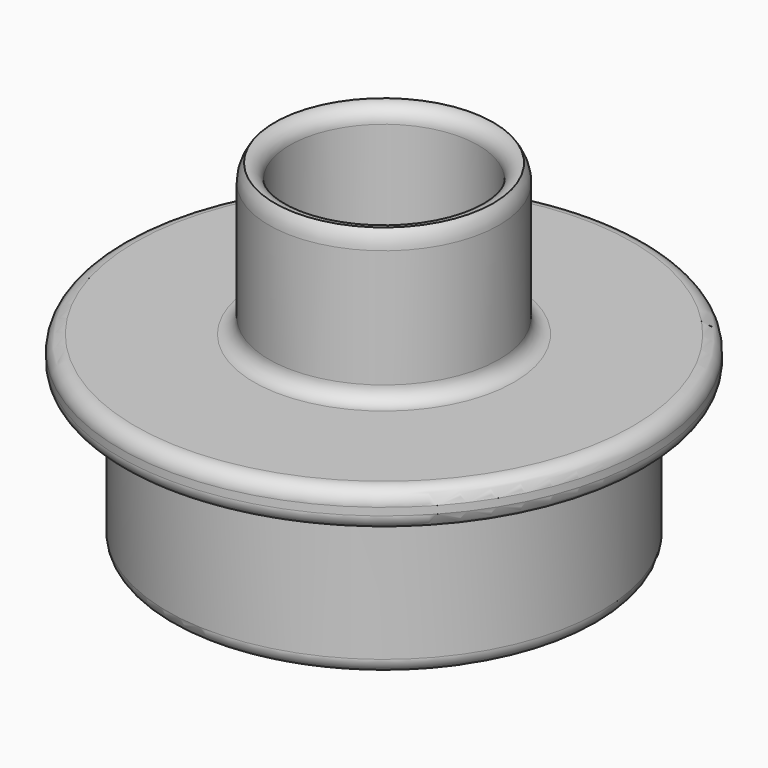
from build123d import *

# Parameters (mm, degrees)
F0_R     = 44.45
F1_DEPTH = 6.35
F2_R     = 36.5125
F3_DEPTH = 25.4
F4_R     = 19.3675
F5_DEPTH = 25.4
F6_R     = 15.875
F7_DEPTH = 31.75
F8_R     = 28.575
F9_DEPTH = 25.4
F10_R    = 2.54


# Not quite as in the source:
# - a fillet or chamfer that OpenCascade refuses, or shapes differently, is made with other operations: its cross-section is extruded or revolved along the edge and cut away or added


with BuildPart() as f1:
    # F0 (on Top) → F1 (new body)
    with BuildSketch(Plane.XY):
        Circle(F0_R)
    extrude(amount=F1_DEPTH)

    # F2 (on face) → F3 (join)
    with BuildSketch(Plane(origin=(0, 0, 0), x_dir=(1, 0, 0), z_dir=(0, 0, -1))):
        Circle(F2_R)
    extrude(amount=F3_DEPTH)

    # F4 (on face) → F5 (join)
    with BuildSketch(Plane.XY.offset(6.35)):
        Circle(F4_R)
    extrude(amount=F5_DEPTH)

    # F6 (on face) → F7 (cut, through all)
    with BuildSketch(Plane.XY.offset(31.75)):
        Circle(F6_R)
    extrude(amount=-F7_DEPTH, mode=Mode.SUBTRACT)

    # F8 (on face) → F9 (cut, through all)
    with BuildSketch(Plane(origin=(0, 0, -25.4), x_dir=(1, 0, 0), z_dir=(0, 0, -1))):
        Circle(F8_R)
    extrude(amount=-F9_DEPTH, mode=Mode.SUBTRACT)

    # F10
    f10_edges = [f1.edges().sort_by_distance(p)[0] for p in [
        (-36.5125, 0, -25.4),
        (-28.575, 0, -25.4),
        (-15.875, 0, 0),
        (-15.875, 0, 31.75),
        (-36.5125, 0, 0),
        (-44.45, 0, 0),
        (-44.45, 0, 6.35),
        (-19.3675, 0, 6.35),
    ]]
    fillet(f10_edges, radius=F10_R)

    # F11: fillet of radius 5.08 on 1 edges, made by hand

    # F11_s1 → F11_t2 (revolve, cut)
    with BuildSketch(Plane.XZ):
        with BuildLine():
            ThreePointArc((19.3675, 28.7885571506), (19.1235159222, 30.3439831373), (18.415, 31.75))
            Line((18.415, 31.75), (19.3675, 31.75))
            Line((19.3675, 31.75), (19.3675, 28.7885571506))
        make_face()
    revolve(axis=Axis((0, 0, 31.75), (0, 0, 1)), mode=Mode.SUBTRACT)


solid = f1.part
